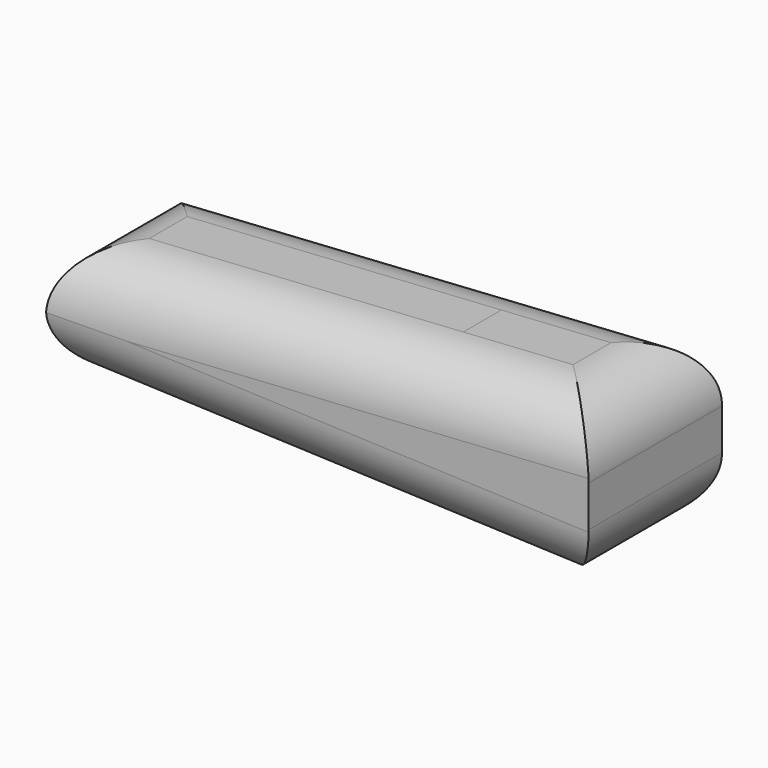
from build123d import *

# Parameters (mm, degrees)
F1_DEPTH      = 7.112
F1_DEPTH_BACK = 7.112
F2_T1_DEPTH   = 38.654431888
F2_T3_DEPTH   = 71.8161099821
F2_T5_DEPTH   = 40.6320472649
F2_T7_DEPTH   = 71.8736907455
F2_T9_DEPTH   = 38.0679604185
F2_T11_DEPTH  = 41.2815855973


# Not quite as in the source:
# - a fillet or chamfer that OpenCascade refuses, or shapes differently, is made with other operations: its cross-section is extruded or revolved along the edge and cut away or added


with BuildPart() as f1:
    # F0 (on Front) → F1 (new body, two sides)
    with BuildSketch(Plane.XZ) as f1_sk:
        Polygon((0, 7.673737593), (-14.7832315415, 6.7385453665), (-14.7832315415, -5.9697437044), (0, -6.5452465788), align=None)
        Polygon((-14.7832315415, 6.7385453665), (-46.3809780777, 4.7396612354), (-46.3809780777, -4.7396612354), (-14.7832315415, -5.9697437044), align=None)
    extrude(amount=F1_DEPTH)
    extrude(f1_sk.sketch, amount=-F1_DEPTH_BACK)

    # F2: fillet of radius 5.08 on 8 edges, made by hand

    # F2_s2 → F2_t1 (cut)
    with BuildSketch(Plane.XZ.offset(-19.327215944)):
        with BuildLine():
            ThreePointArc((-46.3809780777, 0.1464251422), (-44.9622803199, -3.37511797), (-41.4985899316, -4.9297298549))
            Line((-41.4985899316, -4.9297298549), (-46.3809780777, -4.7396612354))
            Line((-46.3809780777, -4.7396612354), (-46.3809780777, 0.1464251422))
        make_face()
    extrude(amount=F2_T1_DEPTH, mode=Mode.SUBTRACT)

    # F2_s4 → F2_t3 (cut)
    with BuildSketch(Plane(origin=(-58.8169483786, 0, 2.2897106602), x_dir=(0, 1, 0), z_dir=(0.9992431097, 0, -0.0388999712))):
        with BuildLine():
            ThreePointArc((-7.112, -1.460292545), (-5.6241024484, -5.0523949934), (-2.032, -6.540292545))
            Line((-2.032, -6.540292545), (-7.112, -6.540292545))
            Line((-7.112, -6.540292545), (-7.112, -1.460292545))
        make_face()
        with BuildLine():
            ThreePointArc((7.112, -1.460292545), (5.6241024484, -5.0523949934), (2.032, -6.540292545))
            Line((2.032, -6.540292545), (7.112, -6.540292545))
            Line((7.112, -6.540292545), (7.112, -1.460292545))
        make_face()
    extrude(amount=F2_T3_DEPTH, mode=Mode.SUBTRACT)

    # F2_s6 → F2_t5 (cut)
    with BuildSketch(Plane.XZ.offset(-20.3160236325)):
        with BuildLine():
            ThreePointArc((0, -1.2636371258), (-1.5584568878, -4.924939368), (-5.2776118539, -6.3397921229))
            Line((-5.2776118539, -6.3397921229), (0, -6.5452465788))
            Line((0, -6.5452465788), (0, -1.2636371258))
        make_face()
    extrude(amount=F2_T5_DEPTH, mode=Mode.SUBTRACT)

    # F2_s8 → F2_t7 (cut)
    with BuildSketch(Plane(origin=(13.1581724385, 0, 0.8323904381), x_dir=(0, 1, 0), z_dir=(-0.9980050505, 0, -0.063134137))):
        with BuildLine():
            ThreePointArc((-2.032, -7.6584288737), (-5.6241024484, -6.1705313222), (-7.112, -2.5784288737))
            Line((-7.112, -2.5784288737), (-7.112, -7.6584288737))
            Line((-7.112, -7.6584288737), (-2.032, -7.6584288737))
        make_face()
        with BuildLine():
            ThreePointArc((7.112, -2.5784288737), (5.6241024484, -6.1705313222), (2.032, -7.6584288737))
            Line((2.032, -7.6584288737), (7.112, -7.6584288737))
            Line((7.112, -7.6584288737), (7.112, -2.5784288737))
        make_face()
    extrude(amount=F2_T7_DEPTH, mode=Mode.SUBTRACT)

    # F2_s10 → F2_t9 (cut)
    with BuildSketch(Plane.XZ.offset(-19.0339802092)):
        with BuildLine():
            ThreePointArc((-46.3809780777, -0.0291308483), (-45.0047373026, 3.4477308981), (-41.6216994935, 5.040734808))
            Line((-41.6216994935, 5.040734808), (-46.3809780777, 4.7396612354))
            Line((-46.3809780777, 4.7396612354), (-46.3809780777, -0.0291308483))
        make_face()
    extrude(amount=F2_T9_DEPTH, mode=Mode.SUBTRACT)

    # F2_s12 → F2_t11 (cut)
    with BuildSketch(Plane.XZ.offset(-20.6407927986)):
        with BuildLine():
            ThreePointArc((0, 2.2622204735), (-1.6031382536, 5.9659796985), (-5.4007214159, 7.3320861299))
            Line((-5.4007214159, 7.3320861299), (0, 7.673737593))
            Line((0, 7.673737593), (0, 2.2622204735))
        make_face()
    extrude(amount=F2_T11_DEPTH, mode=Mode.SUBTRACT)


solid = f1.part
